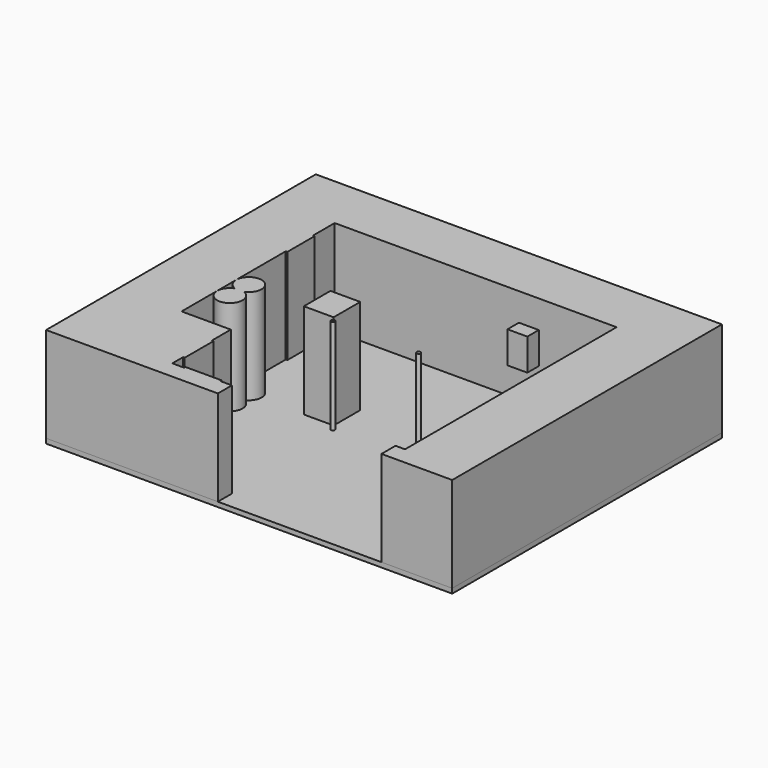
from build123d import *

# Parameters (mm, degrees)
F1_DEPTH = 3048
F0_R     = 63.5
F0_W     = 952.929854393
F0_H     = 1064.3113255501
F2_W     = 12989.7775650024
F2_H     = 10782.4106216431
F3_DEPTH = 152.4
F4_W     = 635
F4_H     = 1016
F5_DEPTH = 457.2


with BuildPart() as f1:
    # F0 (on Top) → F1 (new body)
    with BuildSketch(Plane.XY):
        Polygon((-4497.5893844604, 2806.8917998496), (-4497.5893844604, 3670.4917998496), (1395.2106155395, 3670.4917998496), (2030.2106155395, 3670.4917998496), (4519.4106155395, 3670.4917998496), (4519.4106155396, -4787.7082001504), (4214.6106155396, -4787.7082001504), (4214.6106155396, -5348.7229347229), (6477.6792526245, -5348.7229347229), (6477.6792526245, 5433.6876869202), (-6512.0983123779, 5433.6876869202), (-6512.0983123779, -4787.7082001504), (-6512.0983123779, -5348.7229347229), (-1017.7893844604, -5348.7229347229), (-1017.7893844604, -4787.7082001504), (-1398.7893844604, -4787.7082001504), (-1398.7893844604, -4736.9082001504), (-2541.7893844604, -4736.9082001504), (-2541.7893844604, -4787.7082001504), (-2922.7893844604, -4787.7082001504), (-2922.7893844604, -4355.9082001504), (-2871.9893844604, -4355.9082001504), (-2871.9893844604, -3212.9082001504), (-2922.7893844604, -3212.9082001504), (-2922.7893844604, -2450.9082001504), (-4497.5893844604, -2450.9082001504), (-4497.5893844604, -1434.9082001504), (-4497.5893844604, -1028.5082001504), (-4497.5893844604, -266.5082001504), (-4497.5893844604, 139.8917998496), (-4497.5893844604, 1714.6917998496), (-4446.7893844605, 1714.6917998496), (-4446.7893844605, 2806.8917998496), align=None)
    extrude(amount=F1_DEPTH)

    # F4 (on face) → F5 (join)
    with BuildSketch(Plane.XZ.offset(-3670.4917998496)):
        with Locations((1712.7106155396, 1651)):
            Rectangle(F4_W, F4_H)
    extrude(amount=F5_DEPTH)


with BuildPart() as f1b:
    # F0 (on Top) → F1, piece 2 (new body)
    with BuildSketch(Plane.XY):
        with Locations((1522.2106155396, -495.1082001504)):
            Circle(F0_R)
    extrude(amount=F1_DEPTH)


with BuildPart() as f1c:
    # F0 (on Top) → F1, piece 3 (new body)
    with BuildSketch(Plane.XY):
        with Locations((-1811.0886216164, 206.7666947842)):
            Rectangle(F0_W, F0_H)
    extrude(amount=F1_DEPTH)


with BuildPart() as f1d:
    # F0 (on Top) → F1, piece 4 (new body)
    with BuildSketch(Plane.XY):
        with BuildLine():
            ThreePointArc((-3949.7681696446, -647.5082001504), (-3859.1469548287, 67.1342294814), (-4497.5893844604, -266.5082001504))
            ThreePointArc((-4497.5893844604, -266.5082001504), (-4424.8318140922, -498.5506297821), (-4232.6105992763, -647.5082001504))
            ThreePointArc((-4232.6105992763, -647.5082001504), (-4424.8318140922, -796.4657705186), (-4497.5893844604, -1028.5082001504))
            ThreePointArc((-4497.5893844604, -1028.5082001504), (-3859.1469548287, -1362.1506297821), (-3949.7681696446, -647.5082001504))
        make_face()
    extrude(amount=F1_DEPTH)


with BuildPart() as f1e:
    # F0 (on Top) → F1, piece 5 (new body)
    with BuildSketch(Plane.XY):
        with Locations((-1220.9893844604, -495.1082001504)):
            Circle(F0_R)
    extrude(amount=F1_DEPTH)


with BuildPart() as f3:
    # F2 (on face) → F3 (new body)
    with BuildSketch(Plane(origin=(0, 0, 0), x_dir=(1, 0, 0), z_dir=(0, 0, -1))):
        with Locations((-17.2095298767, -42.4823760986)):
            Rectangle(F2_W, F2_H)
    extrude(amount=F3_DEPTH)


solid = Compound([f1.part, f1b.part, f1c.part, f1d.part, f1e.part, f3.part])
